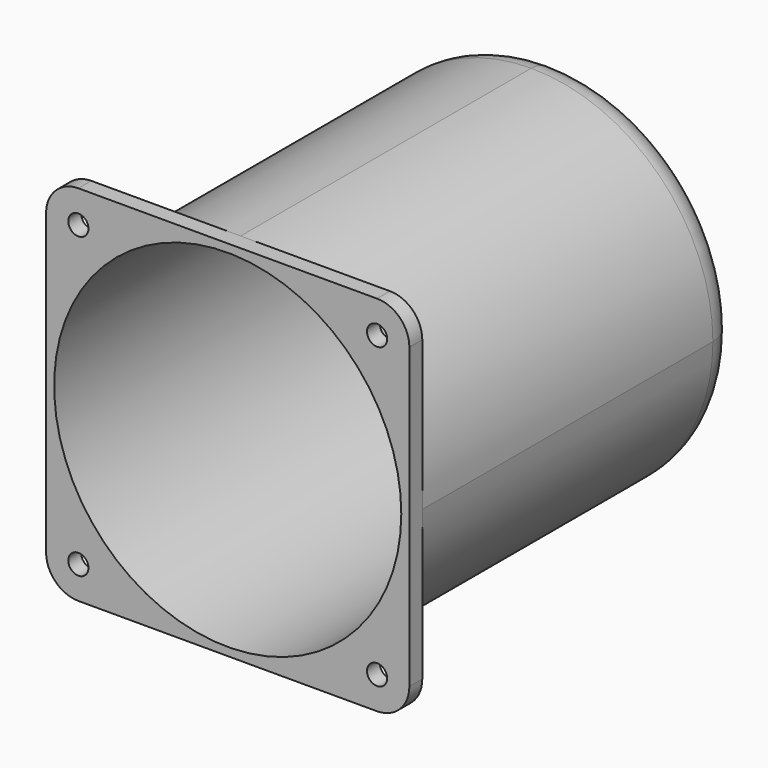
from build123d import *

# Parameters (mm, degrees)
F0_R     = 2.5
F0_R_2   = 43
F1_DEPTH = 4
F2_DEPTH = 98
F3_DEPTH = 94
F4_R     = 8


with BuildPart() as f1:
    # F0 (on Front) → F1 (new body)
    with BuildSketch(Plane.XZ):
        with BuildLine():
            ThreePointArc((0, 45), (31.819805, 31.819805), (45, 0))
            Line((45, 0), (45, 45))
            Line((45, 45), (0, 45))
        make_face()
        with Locations((37, 37)):
            Circle(F0_R, mode=Mode.SUBTRACT)
        with BuildLine():
            Line((-45, 45), (-45, 0))
            ThreePointArc((-45, 0), (-31.819805, 31.819805), (0, 45))
            Line((0, 45), (-45, 45))
        make_face()
        with Locations((-37, 37)):
            Circle(F0_R, mode=Mode.SUBTRACT)
        with BuildLine():
            Line((-45, 0), (-45, -45))
            Line((-45, -45), (0, -45))
            ThreePointArc((0, -45), (-31.819805, -31.819805), (-45, 0))
        make_face()
        with Locations((-37, -37)):
            Circle(F0_R, mode=Mode.SUBTRACT)
        with BuildLine():
            ThreePointArc((45, 0), (31.819805, -31.819805), (0, -45))
            Line((0, -45), (45, -45))
            Line((45, -45), (45, 0))
        make_face()
        with Locations((37, -37)):
            Circle(F0_R, mode=Mode.SUBTRACT)
        with BuildLine():
            ThreePointArc((-45, 0), (-31.819805, -31.819805), (0, -45))
            ThreePointArc((0, -45), (31.819805, -31.819805), (45, 0))
            ThreePointArc((45, 0), (31.819805, 31.819805), (0, 45))
            ThreePointArc((0, 45), (-31.819805, 31.819805), (-45, 0))
        make_face()
        Circle(F0_R_2, mode=Mode.SUBTRACT)
    extrude(amount=F1_DEPTH)

    # F0 (on Front) → F2 (join)
    with BuildSketch(Plane.XZ):
        with BuildLine():
            ThreePointArc((-45, 0), (-31.819805, -31.819805), (0, -45))
            ThreePointArc((0, -45), (31.819805, -31.819805), (45, 0))
            ThreePointArc((45, 0), (31.819805, 31.819805), (0, 45))
            ThreePointArc((0, 45), (-31.819805, 31.819805), (-45, 0))
        make_face()
        Circle(F0_R_2, mode=Mode.SUBTRACT)
        Circle(F0_R_2)
    extrude(amount=-F2_DEPTH)

    # F0 (on Front) → F3 (cut)
    with BuildSketch(Plane.XZ):
        Circle(F0_R_2)
    extrude(amount=-F3_DEPTH, mode=Mode.SUBTRACT)

    # F4
    f4_edges = [f1.edges().sort_by_distance(p)[0] for p in [
        (0, 98, 45),
        (45, -2, 45),
        (45, -2, -45),
        (-45, -2, -45),
        (-45, -2, 45),
    ]]
    fillet(f4_edges, radius=F4_R)


solid = f1.part
